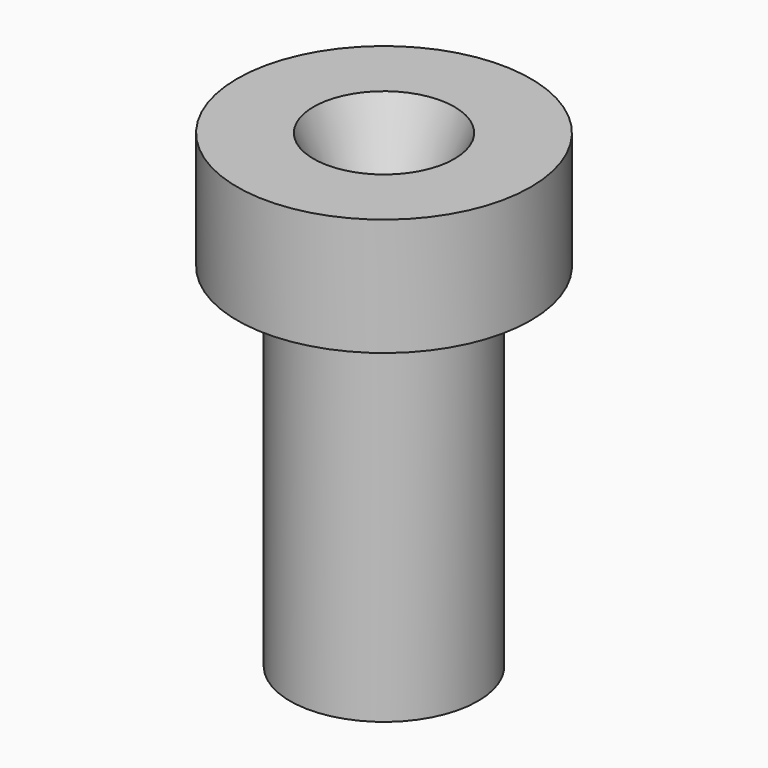
from build123d import *

# Parameters (mm, degrees)
F0_R     = 8
F1_DEPTH = 30
F2_R     = 2
F3_DEPTH = 30
F4_R     = 12.5
F4_R_2   = 8
F4_R_3   = 2
F5_DEPTH = 10
F6_SIZE2 = 9.99999
F6_SIZE  = 3.99999


# Not quite as in the source:
# - a fillet or chamfer is up to 0.001 mm smaller than in the source, because OpenCascade refuses the exact size


with BuildPart() as f1:
    # F0 (on Top) → F1 (new body)
    with BuildSketch(Plane.XY):
        Circle(F0_R)
    extrude(amount=-F1_DEPTH)

    # F2 (on face) → F3 (cut)
    with BuildSketch(Plane.XY):
        Circle(F2_R)
    extrude(amount=-F3_DEPTH, mode=Mode.SUBTRACT)


with BuildPart() as f5:
    # F4 (on face) → F5 (new body)
    with BuildSketch(Plane.XY):
        Circle(F4_R)
        Circle(F4_R_2, mode=Mode.SUBTRACT)
        Circle(F4_R_2)
        Circle(F4_R_3, mode=Mode.SUBTRACT)
    extrude(amount=F5_DEPTH)

    # F6 (size 4 and 10 in the source; OpenCascade refuses exactly that, so slightly less here)
    f6_edges = [f5.edges().sort_by_distance(p)[0] for p in [
        (-2, 0, 10),
    ]]
    f6_side = f5.faces().sort_by_distance((-12.146447, 0, 10))[0]
    chamfer(f6_edges, length=F6_SIZE, length2=F6_SIZE2, reference=f6_side)


solid = Compound([f1.part, f5.part])
